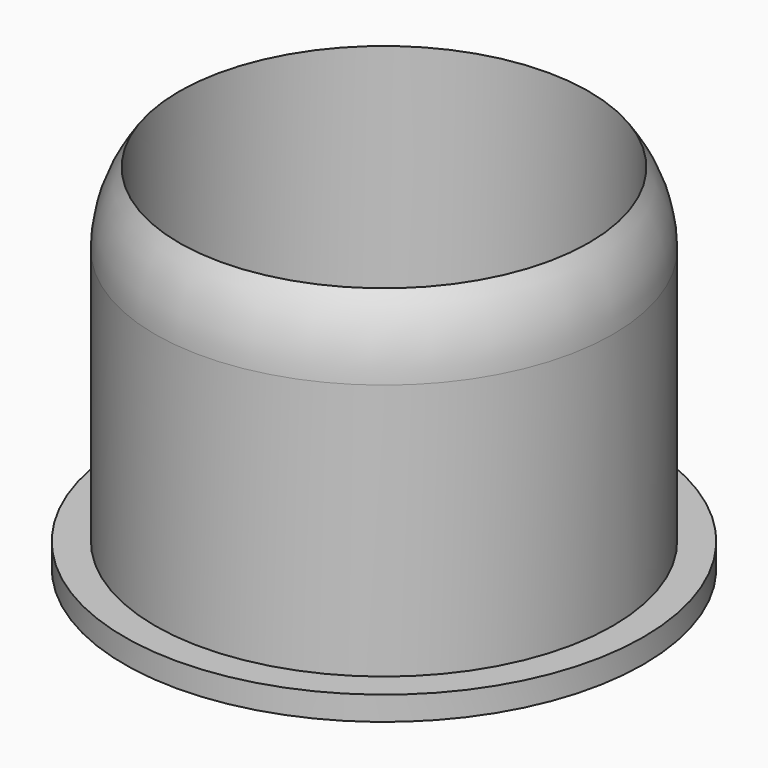
from build123d import *

# Parameters (mm, degrees)
F0_R     = 9.525
F1_DEPTH = 12.7
F2_T     = -1
F3_DEPTH = 1
F4_R     = 10.795
F4_R_2   = 9.525
F5_DEPTH = 1


# Not quite as in the source:
# - a fillet or chamfer that OpenCascade refuses, or shapes differently, is made with other operations: its cross-section is extruded or revolved along the edge and cut away or added


with BuildPart() as f1:
    # F0 (on Top) → F1 (new body)
    with BuildSketch(Plane.XY):
        Circle(F0_R)
    extrude(amount=F1_DEPTH)

    # F2
    f2_openings = [f1.faces().sort_by_distance(p)[0] for p in [
        (0, 0, 12.7),
    ]]
    offset(amount=F2_T, openings=f2_openings)

    # F3 (add): a face of the model
    f3_faces = [f1.faces().sort_by_distance(p)[0] for p in [
        (0, 0, 0),
    ]]
    extrude(f3_faces, amount=F3_DEPTH)

    # F6: fillet of radius 5.08 on 1 edges, made by hand

    # F6_s1 → F6_t2 (revolve, cut)
    with BuildSketch(Plane.XZ):
        with BuildLine():
            ThreePointArc((9.525, 9.6734508099), (9.2685256815, 11.267188555), (8.525, 12.7))
            Line((8.525, 12.7), (9.525, 12.7))
            Line((9.525, 12.7), (9.525, 9.6734508099))
        make_face()
    revolve(axis=Axis((0, 0, 12.7), (0, 0, 1)), mode=Mode.SUBTRACT)


with BuildPart() as f5:
    # F4 (on face) → F5 (new body)
    with BuildSketch(Plane(origin=(0, 0, -1), x_dir=(1, 0, 0), z_dir=(0, 0, -1))):
        Circle(F4_R)
        Circle(F4_R_2, mode=Mode.SUBTRACT)
        Circle(F4_R_2)
    extrude(amount=F5_DEPTH)


solid = Compound([f1.part, f5.part])
